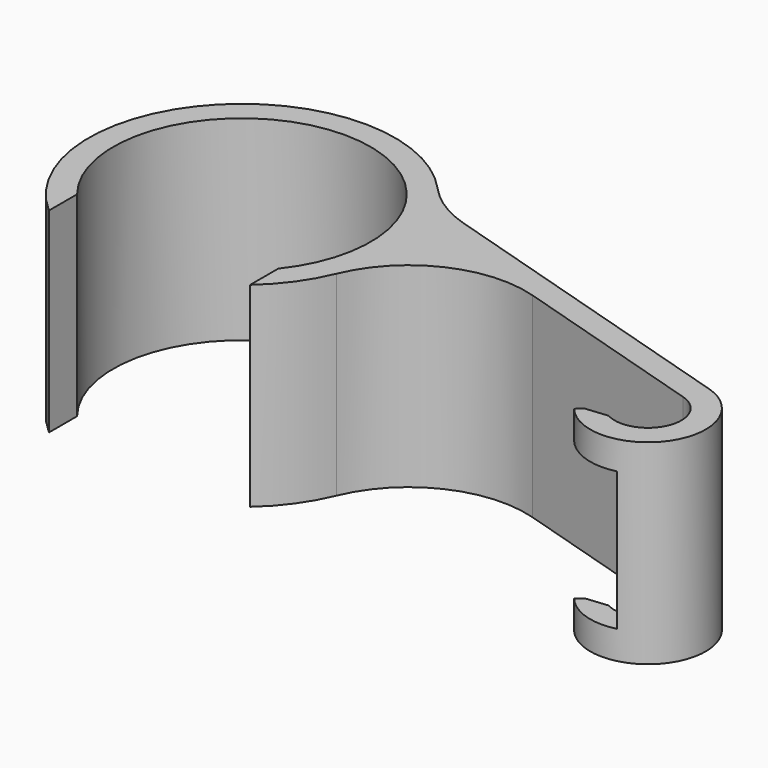
from build123d import *

# Parameters (mm, degrees)
F1_DEPTH    = 25.4
F2_R        = 15.24
F3_T1_DEPTH = 36.0903109365
F4_W        = 3.5194646057
F4_H        = 9.0122472823
F4_W_2      = 2.8517952656
F4_W_3      = 4.2412726252
F5_DEPTH    = 25.4


# Not quite as in the source:
# - a fillet or chamfer that OpenCascade refuses, or shapes differently, is made with other operations: its cross-section is extruded or revolved along the edge and cut away or added


with BuildPart() as f1:
    # F0 (on Top) → F1 (new body)
    with BuildSketch(Plane.XY):
        with BuildLine():
            ThreePointArc((-13.0763784004, -10.4391818642), (0, 16.73225), (13.0763784004, -10.4391818642))
            Line((13.0763784004, -10.4391818642), (13.0763784004, -15.0102275297))
            ThreePointArc((13.0763784004, -15.0102275297), (19.2516474294, -5.0668208785), (18.7713860197, 6.6282478426))
            Line((18.7713860197, 6.6282478426), (62.8066707781, -6.8086651928))
            ThreePointArc((62.8066707781, -6.8086651928), (65.147620689, -13.3496506564), (58.2099580532, -13.7148553544))
            Line((58.2099580532, -13.7148553544), (55.7661979944, -15.7418387719))
            ThreePointArc((55.7661979944, -15.7418387719), (67.7906892269, -15.1088589169), (63.7333095074, -3.7718962412))
            Line((63.7333095074, -3.7718962412), (16.9015827692, 10.5183222263))
            ThreePointArc((16.9015827692, 10.5183222263), (-12.9067718767, 15.1563136113), (-13.0763784004, -15.0102275297))
            Line((-13.0763784004, -15.0102275297), (-13.0763784004, -10.4391818642))
        make_face()
    extrude(amount=F1_DEPTH)

    # F2
    f2_edges = [f1.edges().sort_by_distance(p)[0] for p in [
        (16.901583, 10.518322, 12.7),
        (18.771386, 6.628248, 12.7),
    ]]
    fillet(f2_edges, radius=F2_R)

    # F3: chamfer of 2.54 on 1 edges, made by hand

    # F3_s2 → F3_t1 (cut)
    with BuildSketch(Plane.XY.offset(-5.3451554683)):
        with BuildLine():
            Line((59.4681740413, -14.7511998168), (56.6296179231, -15.0256727671))
            Line((56.6296179231, -15.0256727671), (58.2099580532, -13.7148553544))
            ThreePointArc((58.2099580532, -13.7148553544), (58.8184317915, -14.3160957873), (59.4681740413, -14.7511998168))
        make_face()
    extrude(amount=F3_T1_DEPTH, mode=Mode.SUBTRACT)

    # F4 (on face) → F5 (cut)
    with BuildSketch(Plane(origin=(1.9640154801, -20.3115394411, 0), x_dir=(-0.9953576095, -0.0962456715, 0), z_dir=(-0.0962456715, 0.9953576095, 0))):
        with Locations((-59.5320927234, 8.1938763589)):
            Rectangle(F4_W, F4_H)
        with Locations((-59.5320927234, 17.2061236411)):
            Rectangle(F4_W, F4_H)
        with Locations((-56.3464627878, 17.2061236411)):
            Rectangle(F4_W_2, F4_H)
        with Locations((-56.3464627878, 8.1938763589)):
            Rectangle(F4_W_2, F4_H)
        with Locations((-52.7999288424, 8.1938763589)):
            Rectangle(F4_W_3, F4_H)
        with Locations((-52.7999288424, 17.2061236411)):
            Rectangle(F4_W_3, F4_H)
    extrude(amount=-F5_DEPTH, mode=Mode.SUBTRACT)


solid = f1.part
